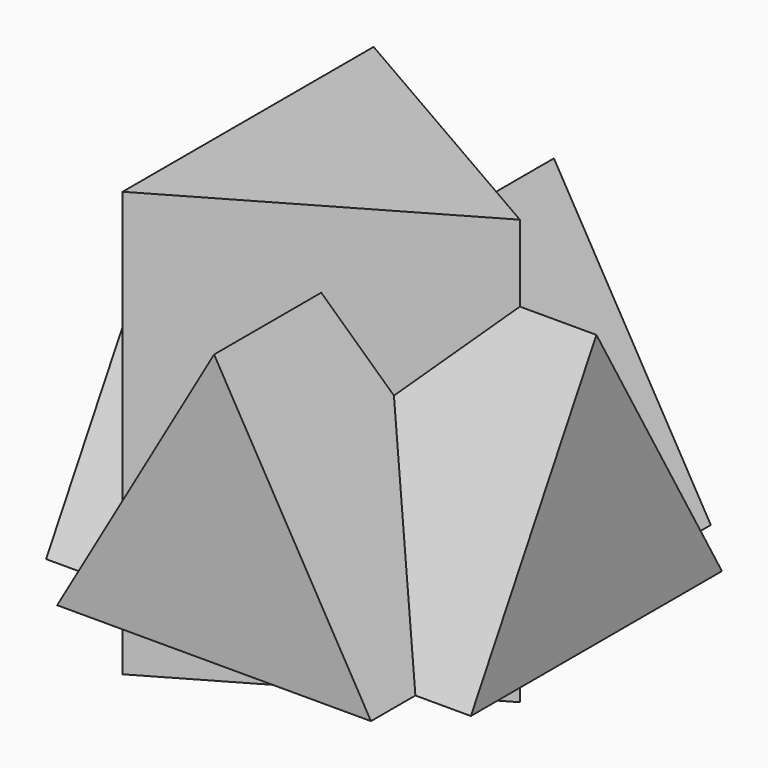
from build123d import *

# Parameters (mm, degrees)
F1_DEPTH = 50.8
F2_DEPTH = 50.8
F3_COUNT = 2
F3_ANGLE = 90
F4_COUNT = 2
F4_ANGLE = 90


# Not quite as in the source:
# - ends of sketch curves that miss each other by under 0.0002 mm in the source are joined
# - a feature names something its author has since deleted; it is built from what else it names


with BuildPart() as f1:
    # F0 (on Right) → F1 (new body)
    with BuildSketch(Plane.YZ):
        Polygon((-6.4567620866, -15.2991628274), (31.070278409, -15.2991628274), (12.3067581612, 17.2002075706), (-6.4567620866, 17.2002075706), align=None)
        Polygon((-43.9838025822, -15.2991628274), (-6.4567620866, -15.2991628274), (-6.4567620866, 17.2001371726), (-25.2202823344, 17.2002075706), align=None)
        Polygon((-25.2202823344, 17.2002075706), (-6.4567620866, 17.2001371726), (-6.4567620866, 49.6995779686), align=None)
        Polygon((-6.4567620866, 17.2002075706), (12.3067581612, 17.2002075706), (-6.4567620866, 49.6995779686), align=None)
    extrude(amount=F1_DEPTH)

    # F2 (add): a face of the model
    f2_faces = [f1.faces().sort_by_distance(p)[0] for p in [
        (0, -6.4567620866, 6.3670841046),
    ]]
    extrude(f2_faces, amount=F2_DEPTH)


with BuildPart() as f3_1:
    # F3: instance of F1
    add(f1.part.rotate(Axis((0, -6.4567620866, 17.2002075706), (0, 1, 0)), 1 * F3_ANGLE / (F3_COUNT - 1)))


with BuildPart() as f4_1:
    # F4: instance of F1
    add(f1.part.rotate(Axis((0, -6.4567620866, 17.2002075706), (0, 0, -1)), 1 * F4_ANGLE / (F4_COUNT - 1)))


solid = Compound([f1.part, f3_1.part, f4_1.part])
